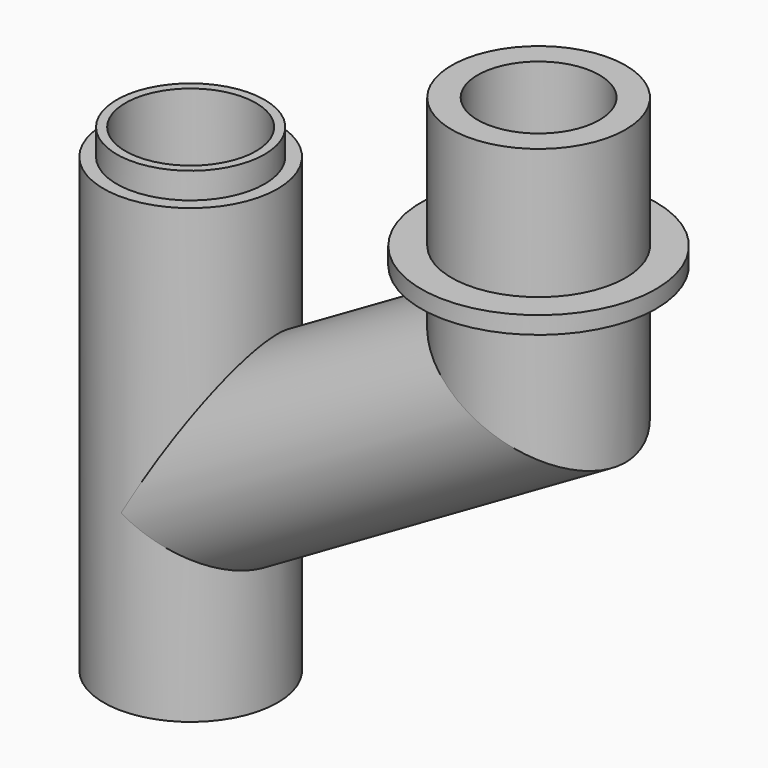
from build123d import *

# Parameters (mm, degrees)
F1_R      = 20
F4_R      = 17.55
F5_DEPTH  = 30
F6_R      = 15
F7_DEPTH  = 110.001
F8_R      = 20
F8_R_2    = 17
F9_DEPTH  = 6
F10_R     = 14
F12_R     = 27
F12_R_2   = 20
F13_DEPTH = 2
F14_DEPTH = 32
F15_R     = 14
F16_DEPTH = 34


with BuildPart() as f2:
    # F2: sweep along a path in F0
    with BuildLine(Plane.XZ) as f2_path:
        Line((0, 0), (0, -70))
        Line((0, -70), (0, -110))
    # F1 (on Top) → F2 (sweep)
    with BuildSketch(Plane.XY):
        Circle(F1_R)
    sweep(path=f2_path.line)

    # F3: sweep along a path in F0
    with BuildLine(Plane.XZ) as f3_path:
        Line((80, 0), (80, -23.8119784648))
        Line((80, -23.8119784648), (0, -70))
    # F1 (on Top) → F3 (sweep)
    with BuildSketch(Plane.XY):
        with Locations((80, 0)):
            Circle(F1_R)
    sweep(path=f3_path.line, transition=Transition.RIGHT)

    # F4 (on face) → F5 (cut)
    with BuildSketch(Plane(origin=(0, 0, -110), x_dir=(1, 0, 0), z_dir=(0, 0, -1))):
        Circle(F4_R)
    extrude(amount=-F5_DEPTH, mode=Mode.SUBTRACT)

    # F6 (on face) → F7 (cut, through all)
    with BuildSketch(Plane.XY):
        Circle(F6_R)
    extrude(amount=-F7_DEPTH, mode=Mode.SUBTRACT)

    # F8 (on face) → F9 (cut)
    with BuildSketch(Plane.XY):
        Circle(F8_R)
        Circle(F8_R_2, mode=Mode.SUBTRACT)
    extrude(amount=-F9_DEPTH, mode=Mode.SUBTRACT)

    # F11: sweep along a path in F0
    with BuildLine(Plane.XZ) as f11_path:
        Line((80, 0), (80, -23.8119784648))
        Line((80, -23.8119784648), (0, -70))
    # F10 (on face) → F11 (sweep, cut)
    with BuildSketch(Plane.XY):
        with Locations((80, 0)):
            Circle(F10_R)
    sweep(path=f11_path.line, transition=Transition.RIGHT, mode=Mode.SUBTRACT)

    # F12 (on face) → F13 (join, symmetric)
    with BuildSketch(Plane.XY):
        with Locations((80, 0)):
            Circle(F12_R)
        with Locations((80, 0)):
            Circle(F12_R_2, mode=Mode.SUBTRACT)
    extrude(amount=F13_DEPTH, both=True)

    # F1 (on Top) → F14 (join)
    with BuildSketch(Plane.XY):
        with Locations((80, 0)):
            Circle(F1_R)
    extrude(amount=F14_DEPTH)

    # F15 (on face) → F16 (cut)
    with BuildSketch(Plane.XY.offset(32)):
        with Locations((80, 0)):
            Circle(F15_R)
    extrude(amount=-F16_DEPTH, mode=Mode.SUBTRACT)


solid = f2.part
